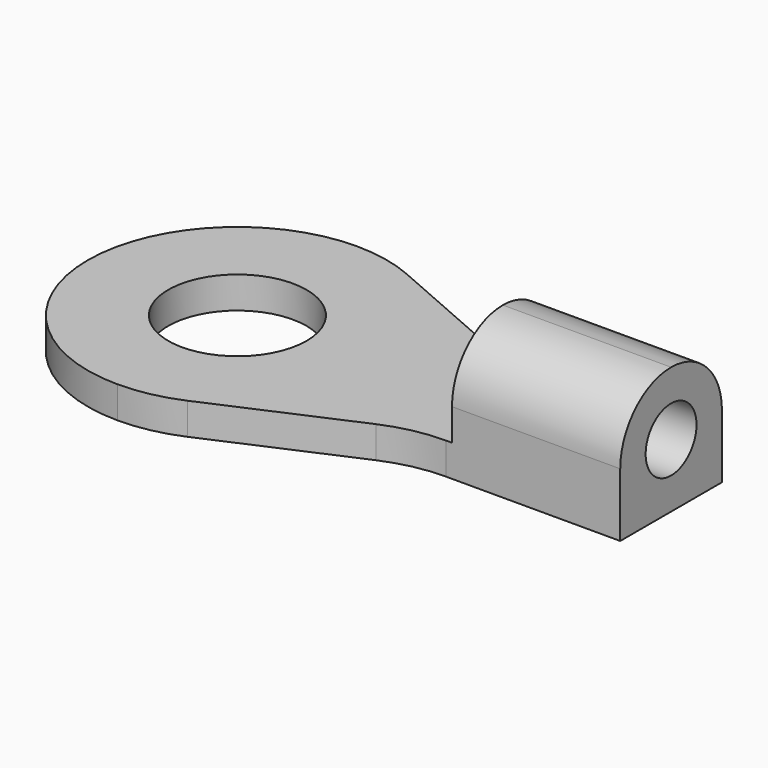
from build123d import *

# Parameters (mm, degrees)
F0_R     = 1.85
F1_DEPTH = 0.85
F2_W     = 4.5
F2_H     = 3.4
F3_DEPTH = 2.55
F4_R     = 1.69999
F5_R     = 0.85
F6_DEPTH = 25


# Not quite as in the source:
# - a fillet or chamfer is up to 0.001 mm smaller than in the source, because OpenCascade refuses the exact size


with BuildPart() as f1:
    # F0 (on Top) → F1 (new body)
    with BuildSketch(Plane.XY):
        with BuildLine():
            Line((10.9356666081, 2.3), (15.6, 2.3))
            Line((15.6, 2.3), (15.6, 5.7))
            Line((15.6, 5.7), (10.9356666081, 5.7))
            ThreePointArc((10.9356666081, 5.7), (10.117660762, 5.7845349656), (9.3342299639, 6.0345667821))
            Line((9.3342299639, 6.0345667821), (5.6014366442, 7.6654332179))
            ThreePointArc((5.6014366442, 7.6654332179), (4.8180058461, 7.9154650344), (4, 8))
            ThreePointArc((4, 8), (1.1715728753, 6.8284271247), (0, 4))
            ThreePointArc((0, 4), (1.1715728753, 1.1715728753), (4, 0))
            ThreePointArc((4, 0), (4.8180058461, 0.0845349656), (5.6014366442, 0.3345667821))
            Line((5.6014366442, 0.3345667821), (9.3342299639, 1.9654332179))
            ThreePointArc((9.3342299639, 1.9654332179), (10.117660762, 2.2154650344), (10.9356666081, 2.3))
        make_face()
        with Locations((4, 4)):
            Circle(F0_R, mode=Mode.SUBTRACT)
    extrude(amount=F1_DEPTH)

    # F2 (on face) → F3 (join)
    with BuildSketch(Plane.XY.offset(0.85)):
        with Locations((13.35, 4)):
            Rectangle(F2_W, F2_H)
    extrude(amount=F3_DEPTH)

    # F4 (radius 1.7 in the source; OpenCascade refuses exactly that, so slightly less here)
    f4_edges = [f1.edges().sort_by_distance(p)[0] for p in [
        (13.35, 5.7, 3.4),
        (13.35, 2.3, 3.4),
    ]]
    fillet(f4_edges, radius=F4_R)

    # F5 (on face) → F6 (cut)
    with BuildSketch(Plane.YZ.offset(15.6)):
        with Locations((4, 1.7)):
            Circle(F5_R)
    extrude(amount=-F6_DEPTH, mode=Mode.SUBTRACT)


solid = f1.part
